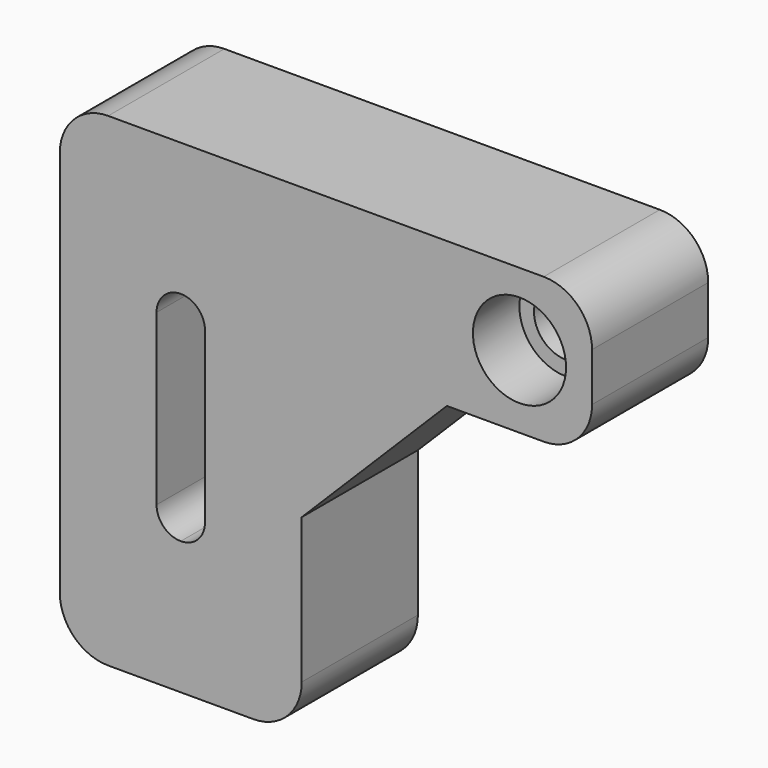
from build123d import *

# Parameters (mm, degrees)
F1_DEPTH       = 30
F3_D           = 13.2
F3_CBORE_D     = 19.25
F3_CBORE_DEPTH = 12
F4_R           = 10
F5_W           = 10
F5_H           = 45
F6_DEPTH       = 30.001
F7_R           = 4.99999


# Not quite as in the source:
# - a fillet or chamfer is up to 0.001 mm smaller than in the source, because OpenCascade refuses the exact size


with BuildPart() as f1:
    # F0 (on Front) → F1 (new body)
    with BuildSketch(Plane.XZ):
        Polygon((0, 100), (0, 0), (50, 0), (50, 40), (80, 70), (110, 70), (110, 100), align=None)
    extrude(amount=-F1_DEPTH)

    # F3 (through all)
    with Locations(Plane.XZ):
        with Locations((95, 85)):
            CounterBoreHole(F3_D / 2, F3_CBORE_D / 2, F3_CBORE_DEPTH)

    # F4
    f4_edges = [f1.edges().sort_by_distance(p)[0] for p in [
        (0, 15, 100),
        (50, 15, 0),
        (110, 15, 70),
        (110, 15, 100),
        (0, 15, 0),
    ]]
    fillet(f4_edges, radius=F4_R)

    # F5 (on face) → F6 (cut, through all)
    with BuildSketch(Plane.XZ):
        with Locations((25, 50)):
            Rectangle(F5_W, F5_H)
    extrude(amount=-F6_DEPTH, mode=Mode.SUBTRACT)

    # F7 (radius 5 in the source; OpenCascade refuses exactly that, so slightly less here)
    f7_edges = [f1.edges().sort_by_distance(p)[0] for p in [
        (20, 15, 72.5),
        (30, 15, 72.5),
        (30, 15, 27.5),
        (20, 15, 27.5),
    ]]
    fillet(f7_edges, radius=F7_R)


solid = f1.part
